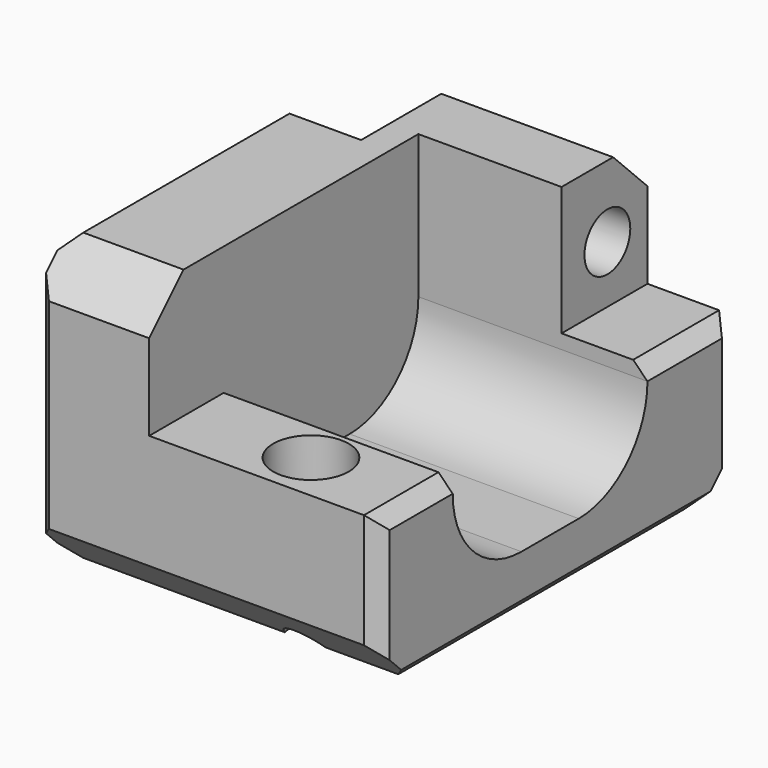
from build123d import *

# Parameters (mm, degrees)
F0_W      = 12
F0_H      = 15.5
F1_DEPTH  = 10
F3_DEPTH  = 4.5
F4_W      = 8.5
F4_H      = 3.5
F5_DEPTH  = 8
F6_R      = 3
F7_SIZE   = 1.5
F9_D      = 2
F9_DEPTH  = 3
F9_TIP    = 0.600860619
F12_W     = 5
F12_H     = 4.5
F13_DEPTH = 3
F14_R     = 3
F16_D     = 2
F18_D     = 1.5
F20_D     = 2.64
F20_DEPTH = 1.624
F20_TIP   = 0.7931360171
F21_SIZE  = 0.5
F23_D     = 2.4
F23_DEPTH = 6
F23_START = 0.2
F23_TIP   = 0.7210327428
F25_D     = 2.4
F25_DEPTH = 6
F25_START = 0.95
F25_TIP   = 0.7210327428


# Not quite as in the source:
# - a feature of the source that left no trace in its solid (it failed there, or was rolled back) is left out


with BuildPart() as f1:
    # F0 (on Top) → F1 (new body)
    with BuildSketch(Plane.XY):
        Rectangle(F0_W, F0_H)
    extrude(amount=F1_DEPTH)

    # F2 (on face) → F3 (cut)
    with BuildSketch(Plane.XY.offset(10)):
        Polygon((-2, -7.75), (6, -7.75), (6, 7.75), (3, 7.75), (3, 4), (-2, 4), align=None)
    extrude(amount=-F3_DEPTH, mode=Mode.SUBTRACT)

    # F4 (on face) → F5 (cut)
    with BuildSketch(Plane.YZ.offset(6)):
        with Locations((-0.25, 3.75)):
            Rectangle(F4_W, F4_H)
    extrude(amount=-F5_DEPTH, mode=Mode.SUBTRACT)

    # F6
    f6_edges = [f1.edges().sort_by_distance(p)[0] for p in [
        (2, 4, 2),
        (2, -4.5, 2),
    ]]
    fillet(f6_edges, radius=F6_R)

    # F7
    f7_edges = [f1.edges().sort_by_distance(p)[0] for p in [
        (-1.5, 7.75, 10),
        (0, -7.75, 0),
        (-4, -7.75, 10),
        (0, 7.75, 0),
    ]]
    chamfer(f7_edges, length=F7_SIZE)

    # F9
    with Locations(Plane(origin=(-6, 0, 0), x_dir=(0, -1, 0), z_dir=(-1, 0, 0))):
        with Locations((0, 6)):
            Hole(F9_D / 2, depth=F9_DEPTH)
            with Locations((0, 0, -(F9_DEPTH + F9_TIP / 2))):  # 118° drill point
                Cone(0, F9_D / 2, F9_TIP, mode=Mode.SUBTRACT)

    # F12 (on face) → F13 (cut)
    with BuildSketch(Plane(origin=(-6, 0, 0), x_dir=(0, -1, 0), z_dir=(-1, 0, 0))):
        with Locations((-5.25, 7.75)):
            Rectangle(F12_W, F12_H)
    extrude(amount=-F13_DEPTH, mode=Mode.SUBTRACT)

    # F14
    f14_edges = [f1.edges().sort_by_distance(p)[0] for p in [
        (-4.5, 2.75, 5.5),
    ]]
    fillet(f14_edges, radius=F14_R)

    # F16 (through all)
    with Locations(Plane(origin=(-3, 0, 0), x_dir=(0, -1, 0), z_dir=(-1, 0, 0))):
        with Locations((-6, 7.5)):
            Hole(F16_D / 2)

    # F18 (through all)
    with Locations(Plane.XY.offset(5.5)):
        with Locations((2.25, -6)):
            Hole(F18_D / 2)

    # F20
    with Locations(Plane.XY.offset(5.5)):
        with Locations((2.25, -6)):
            Hole(F20_D / 2, depth=F20_DEPTH)
            with Locations((0, 0, -(F20_DEPTH + F20_TIP / 2))):  # 118° drill point
                Cone(0, F20_D / 2, F20_TIP, mode=Mode.SUBTRACT)

    # F21
    f21_edges = [f1.edges().sort_by_distance(p)[0] for p in [
        (-6, -1.75, 10),
        (6, -6.125, 5.5),
        (6, 5.875, 5.5),
        (6, 7.75, 3.5),
        (6, 0, 0),
        (-6, 0, 0),
        (-6, -7.75, 5),
        (-6, 7.75, 3.5),
        (6, -7.75, 3.5),
    ]]
    chamfer(f21_edges, length=F21_SIZE)

    # F23
    # its depths count from where the whole tool has entered the part; down to there all is cleared
    with Locations(Plane(origin=(0, 0, 0), x_dir=(1, 0, 0), z_dir=(0, 0, -1)).offset(-F23_START)):
        with Locations((-4.5, 0)):
            Hole(F23_D / 2, depth=F23_DEPTH)
            with Locations((0, 0, -(F23_DEPTH + F23_TIP / 2))):  # 118° drill point
                Cone(0, F23_D / 2, F23_TIP, mode=Mode.SUBTRACT)

    # F25
    # its depths count from where the whole tool has entered the part; down to there all is cleared
    with Locations(Plane(origin=(0, 0, 0), x_dir=(1, 0, 0), z_dir=(0, 0, -1)).offset(-F25_START)):
        with Locations((0, -6)):
            Hole(F25_D / 2, depth=F25_DEPTH)
            with Locations((0, 0, -(F25_DEPTH + F25_TIP / 2))):  # 118° drill point
                Cone(0, F25_D / 2, F25_TIP, mode=Mode.SUBTRACT)


solid = f1.part
